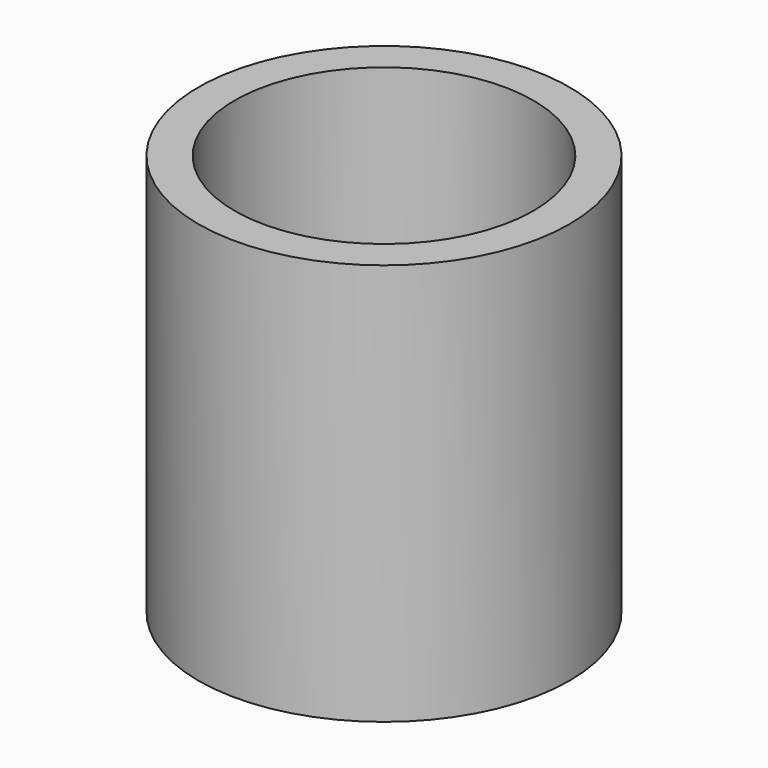
from build123d import *
from build123d import SkipClean  # not in build123d's __all__

# Parameters (mm, degrees)
F0_R     = 18
F0_R_2   = 14.5
F1_DEPTH = 36
F2_R     = 18
F3_DEPTH = 3
F5_DEPTH = 25


with BuildPart() as f1:
    # F0 (on Top) → F1 (new body)
    with BuildSketch(Plane.XY):
        Circle(F0_R)
        Circle(F0_R_2, mode=Mode.SUBTRACT)
    extrude(amount=F1_DEPTH)

    # F2 (on face) → F3 (join)
    with BuildSketch(Plane(origin=(0, 0, 0), x_dir=(1, 0, 0), z_dir=(0, 0, -1))):
        Circle(F2_R)
    extrude(amount=F3_DEPTH)

    # F4 (on face) → F5 (cut)
    with BuildSketch(Plane(origin=(0, 0, -3), x_dir=(1, 0, 0), z_dir=(0, 0, -1))):
        with BuildLine():
            Line((-4.7296723619, 5.8206700086), (-8.8702309022, 11.4703532527))
            ThreePointArc((-8.8702309022, 11.4703532527), (-13.0166882901, 6.388726474), (-14.5, 0))
            Line((-14.5, 0), (-7.5, 0))
            ThreePointArc((-7.5, 0), (-6.7720950493, 3.2231550758), (-4.7296723619, 5.8206700086))
        make_face()
        with BuildLine():
            ThreePointArc((7.5, 0), (3.2231550758, 6.7720950493), (-4.7296723619, 5.8206700086))
            ThreePointArc((-4.7296723619, 5.8206700086), (-6.7720950493, 3.2231550758), (-7.5, 0))
            ThreePointArc((-7.5, 0), (-3.2231550758, -6.7720950493), (4.7296723619, -5.8206700086))
            ThreePointArc((4.7296723619, -5.8206700086), (6.7720950493, -3.2231550758), (7.5, 0))
        make_face()
        with BuildLine():
            Line((14.5, 0), (7.5, 0))
            ThreePointArc((7.5, 0), (6.7720950493, -3.2231550758), (4.7296723619, -5.8206700086))
            Line((4.7296723619, -5.8206700086), (8.8702309022, -11.4703532527))
            ThreePointArc((8.8702309022, -11.4703532527), (13.0166882901, -6.388726474), (14.5, 0))
        make_face()
    with SkipClean():  # cleaning this boolean's faces spoils the solid; the shape is the same uncleaned
        extrude(amount=-F5_DEPTH, mode=Mode.SUBTRACT)


solid = f1.part
